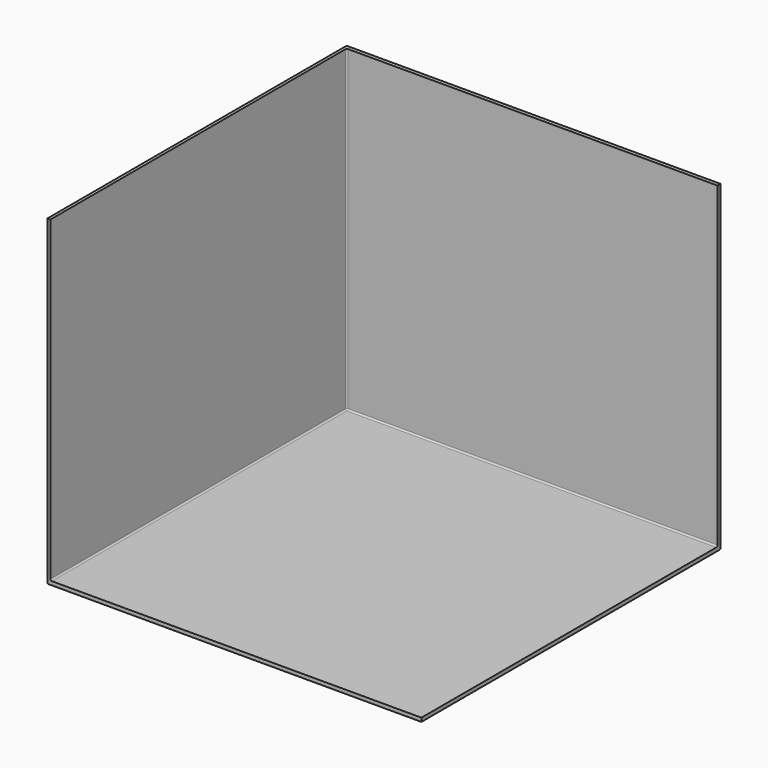
from build123d import *

# Parameters (mm, degrees)
F0_W     = 5
F0_H     = 430
F1_DEPTH = 500
F2_W     = 500
F2_H     = 500
F3_DEPTH = 5
F4_W     = 4
F4_H     = 495
F5_DEPTH = 430
F7_R     = 2


# Not quite as in the source:
# - a feature names something its author has since deleted; it is built from what else it names


with BuildPart() as f1:
    # F0 (on Right) → F1 (new body)
    with BuildSketch(Plane.YZ):
        with Locations((-2.5, 215)):
            Rectangle(F0_W, F0_H)
    extrude(amount=F1_DEPTH)

    # F2 (on Top) → F3 (join)
    with BuildSketch(Plane.XY):
        with Locations((250, -250)):
            Rectangle(F2_W, F2_H)
    extrude(amount=F3_DEPTH)


with BuildPart() as f5:
    # F4 (on face) → F5 (new body, through all)
    with BuildSketch(Plane.XY.offset(430)):
        with Locations((2, -252.5)):
            Rectangle(F4_W, F4_H)
    extrude(amount=-F5_DEPTH)

    # F6: union F1
    add(f1.part)

    # F7
    f7_edges = [f5.edges().sort_by_distance(p)[0] for p in [
        (0, 0, 215),
        (250, 0, 0),
        (0, -250, 0),
        (252, -5, 5),
        (4, -5, 217.5),
        (4, -252.5, 5),
    ]]
    fillet(f7_edges, radius=F7_R)


solid = f5.part
